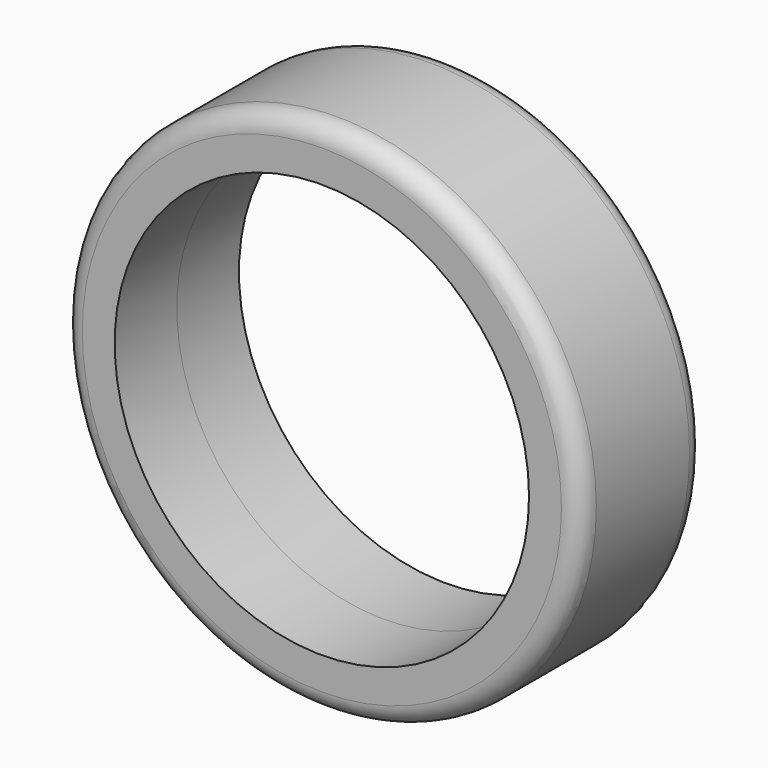
from build123d import *

# Parameters (mm, degrees)
F0_R          = 254
F0_R_2        = 203.2
F2_DEPTH      = 76.2
F2_DEPTH_BACK = 76.2
F3_R          = 19.05


# Not quite as in the source:
# - the program builds the solid bodies; features that only make, move or delete a surface that nothing else refers to are left out


with BuildPart() as f2:
    # F0 (on Front) → F2 (new body, two sides)
    with BuildSketch(Plane.XZ) as f2_sk:
        Circle(F0_R)
        Circle(F0_R_2, mode=Mode.SUBTRACT)
    extrude(amount=F2_DEPTH)
    extrude(f2_sk.sketch, amount=-F2_DEPTH_BACK)

    # F3
    f3_edges = [f2.edges().sort_by_distance(p)[0] for p in [
        (-254, 76.2, 0),
        (-254, -76.2, 0),
    ]]
    fillet(f3_edges, radius=F3_R)


solid = f2.part
